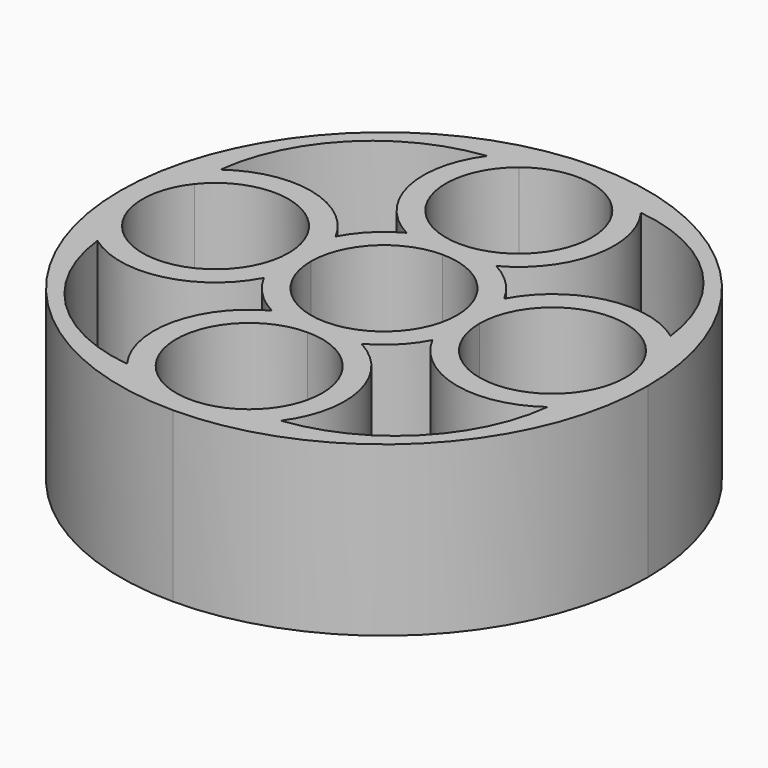
from build123d import *

# Parameters (mm, degrees)
F1_DEPTH = 25.4


# Not quite as in the source:
# - a feature names something its author has since deleted; it is built from what else it names


with BuildPart() as f1:
    # F0 (on Top) → F1 (new body)
    with BuildSketch(Plane.XY):
        with BuildLine():
            ThreePointArc((12.7, -6.7643328429), (11.4395600211, -3.4860169829), (11.0109, 0))
            ThreePointArc((11.0109, 0), (7.785882057, -7.785882057), (0, -11.0109))
            ThreePointArc((0, -11.0109), (3.4860169829, -11.4395600211), (6.7643328429, -12.7))
            ThreePointArc((6.7643328429, -12.7), (10.1746301852, -10.1746301852), (12.7, -6.7643328429))
        make_face()
        with BuildLine():
            ThreePointArc((-11.0109, 0), (-7.785882056, 7.7858820579), (2.7e-09, 11.0109))
            ThreePointArc((2.7e-09, 11.0109), (-3.4860169816, 11.4395600208), (-6.7643328429, 12.7))
            ThreePointArc((-6.7643328429, 12.7), (-10.1746301852, 10.1746301852), (-12.7, 6.7643328429))
            ThreePointArc((-12.7, 6.7643328429), (-11.4395600211, 3.4860169829), (-11.0109, 0))
        make_face()
        with BuildLine():
            ThreePointArc((6.7643328429, 12.7), (3.4860169842, 11.4395600214), (2.7e-09, 11.0109))
            ThreePointArc((2.7e-09, 11.0109), (7.7858820579, 7.785882056), (11.0109, 0))
            ThreePointArc((11.0109, 0), (11.4395600211, 3.4860169829), (12.7, 6.7643328429))
            ThreePointArc((12.7, 6.7643328429), (10.1746301852, 10.1746301852), (6.7643328429, 12.7))
        make_face()
        with BuildLine():
            ThreePointArc((0, -11.0109), (-7.785882057, -7.785882057), (-11.0109, 0))
            ThreePointArc((-11.0109, 0), (-11.4395600211, -3.4860169829), (-12.7, -6.7643328429))
            ThreePointArc((-12.7, -6.7643328429), (-10.1746301852, -10.1746301852), (-6.7643328429, -12.7))
            ThreePointArc((-6.7643328429, -12.7), (-3.4860169829, -11.4395600211), (0, -11.0109))
        make_face()
        with BuildLine():
            ThreePointArc((-6.8403930724, 34.02838), (0, 36.4109), (6.8403930724, 34.02838))
            ThreePointArc((6.8403930724, 34.02838), (9.216102766, 34.090951688), (11.5872617117, 33.9312112173))
            ThreePointArc((11.5872617117, 33.9312112173), (6.4919083282, 38.2413910878), (0, 39.7891))
            ThreePointArc((0, 39.7891), (-6.4919083282, 38.2413910878), (-11.5872617117, 33.9312112173))
            ThreePointArc((-11.5872617117, 33.9312112173), (-9.216102766, 34.090951688), (-6.8403930724, 34.02838))
        make_face()
        with BuildLine():
            ThreePointArc((0, 39.7891), (6.4919083282, 38.2413910878), (11.5872617117, 33.9312112173))
            ThreePointArc((11.5872617117, 33.9312112173), (26.6567838655, 26.6567838655), (33.9312112173, 11.5872617117))
            ThreePointArc((33.9312112173, 11.5872617117), (38.2413910878, 6.4919083282), (39.7891, 0))
            ThreePointArc((39.7891, 0), (28.1351424273, 28.1351424273), (0, 39.7891))
        make_face()
        with BuildLine():
            ThreePointArc((6.8403930724, 34.02838), (9.9135967966, 30.1917134059), (11.0109, 25.4))
            ThreePointArc((11.0109, 25.4), (7.7858820586, 17.6141179447), (4.7e-09, 14.3891))
            ThreePointArc((4.7e-09, 14.3891), (3.4860169852, 13.9604399783), (6.7643328429, 12.7))
            ThreePointArc((6.7643328429, 12.7), (12.3365080254, 17.9934644705), (14.3891, 25.4))
            ThreePointArc((14.3891, 25.4), (13.6707071197, 29.8897623163), (11.5872617117, 33.9312112173))
            ThreePointArc((11.5872617117, 33.9312112173), (9.216102766, 34.090951688), (6.8403930724, 34.02838))
        make_face()
        with BuildLine():
            ThreePointArc((-6.7643328429, 12.7), (-3.4860169806, 13.9604399795), (4.7e-09, 14.3891))
            ThreePointArc((4.7e-09, 14.3891), (-10.3982245629, 21.7782815197), (-6.8403930724, 34.02838))
            ThreePointArc((-6.8403930724, 34.02838), (-9.216102766, 34.090951688), (-11.5872617117, 33.9312112173))
            ThreePointArc((-11.5872617117, 33.9312112173), (-14.0316192263, 22.2125463616), (-6.7643328429, 12.7))
        make_face()
        with BuildLine():
            ThreePointArc((-33.9312112173, 11.5872617117), (-26.6567838655, 26.6567838655), (-11.5872617117, 33.9312112173))
            ThreePointArc((-11.5872617117, 33.9312112173), (-6.4919083282, 38.2413910878), (0, 39.7891))
            ThreePointArc((0, 39.7891), (-28.1351424273, 28.1351424273), (-39.7891, 0))
            ThreePointArc((-39.7891, 0), (-38.2413910878, 6.4919083282), (-33.9312112173, 11.5872617117))
        make_face()
        with BuildLine():
            ThreePointArc((-34.02838, 6.8403930724), (-34.090951688, 9.216102766), (-33.9312112173, 11.5872617117))
            ThreePointArc((-33.9312112173, 11.5872617117), (-38.2413910878, 6.4919083282), (-39.7891, 0))
            ThreePointArc((-39.7891, 0), (-38.2413910878, -6.4919083282), (-33.9312112173, -11.5872617117))
            ThreePointArc((-33.9312112173, -11.5872617117), (-34.090951688, -9.216102766), (-34.02838, -6.8403930724))
            ThreePointArc((-34.02838, -6.8403930724), (-36.4109, 0), (-34.02838, 6.8403930724))
        make_face()
        with BuildLine():
            ThreePointArc((-12.7, -6.7643328429), (-13.9604399789, -3.4860169829), (-14.3891, 0))
            ThreePointArc((-14.3891, 0), (-21.778281522, -10.3982245636), (-34.02838, -6.8403930724))
            ThreePointArc((-34.02838, -6.8403930724), (-34.090951688, -9.216102766), (-33.9312112173, -11.5872617117))
            ThreePointArc((-33.9312112173, -11.5872617117), (-22.2125463616, -14.0316192263), (-12.7, -6.7643328429))
        make_face()
        with BuildLine():
            ThreePointArc((-33.9312112173, -11.5872617117), (-38.2413910878, -6.4919083282), (-39.7891, 0))
            ThreePointArc((-39.7891, 0), (-28.1351424844, -28.1351423702), (-1.615e-07, -39.7891))
            ThreePointArc((-1.615e-07, -39.7891), (-6.4919084002, -38.2413910513), (-11.5872617117, -33.9312112173))
            ThreePointArc((-11.5872617117, -33.9312112173), (-26.6567838655, -26.6567838655), (-33.9312112173, -11.5872617117))
        make_face()
        with BuildLine():
            ThreePointArc((-6.8403930724, -34.02838), (-10.3982245667, -21.7782815309), (-1.89e-08, -14.3891))
            ThreePointArc((-1.89e-08, -14.3891), (-3.486016992, -13.9604399766), (-6.7643328429, -12.7))
            ThreePointArc((-6.7643328429, -12.7), (-14.0316192263, -22.2125463616), (-11.5872617117, -33.9312112173))
            ThreePointArc((-11.5872617117, -33.9312112173), (-9.216102766, -34.090951688), (-6.8403930724, -34.02838))
        make_face()
        with BuildLine():
            ThreePointArc((-11.5872617117, -33.9312112173), (-6.4919084002, -38.2413910513), (-1.615e-07, -39.7891))
            ThreePointArc((-1.615e-07, -39.7891), (6.4919082561, -38.2413911242), (11.5872617117, -33.9312112173))
            ThreePointArc((11.5872617117, -33.9312112173), (9.216102766, -34.090951688), (6.8403930724, -34.02838))
            ThreePointArc((6.8403930724, -34.02838), (0, -36.4109), (-6.8403930724, -34.02838))
            ThreePointArc((-6.8403930724, -34.02838), (-9.216102766, -34.090951688), (-11.5872617117, -33.9312112173))
        make_face()
        with BuildLine():
            ThreePointArc((6.7643328429, -12.7), (3.4860169737, -13.9604399812), (-1.89e-08, -14.3891))
            ThreePointArc((-1.89e-08, -14.3891), (7.7858820503, -17.6141179364), (11.0109, -25.4))
            ThreePointArc((11.0109, -25.4), (9.9135967966, -30.1917134059), (6.8403930724, -34.02838))
            ThreePointArc((6.8403930724, -34.02838), (9.216102766, -34.090951688), (11.5872617117, -33.9312112173))
            ThreePointArc((11.5872617117, -33.9312112173), (13.6707071197, -29.8897623163), (14.3891, -25.4))
            ThreePointArc((14.3891, -25.4), (12.3365080254, -17.9934644705), (6.7643328429, -12.7))
        make_face()
        with BuildLine():
            ThreePointArc((-1.615e-07, -39.7891), (28.1351423702, -28.1351424844), (39.7891, 0))
            ThreePointArc((39.7891, 0), (38.2413910878, -6.4919083282), (33.9312112173, -11.5872617117))
            ThreePointArc((33.9312112173, -11.5872617117), (26.6567838655, -26.6567838655), (11.5872617117, -33.9312112173))
            ThreePointArc((11.5872617117, -33.9312112173), (6.4919082561, -38.2413911242), (-1.615e-07, -39.7891))
        make_face()
        with BuildLine():
            ThreePointArc((39.7891, 0), (38.2413910878, 6.4919083282), (33.9312112173, 11.5872617117))
            ThreePointArc((33.9312112173, 11.5872617117), (34.090951688, 9.216102766), (34.02838, 6.8403930724))
            ThreePointArc((34.02838, 6.8403930724), (35.7982245636, 3.621718478), (36.4109, 0))
            ThreePointArc((36.4109, 0), (35.7982245636, -3.621718478), (34.02838, -6.8403930724))
            ThreePointArc((34.02838, -6.8403930724), (34.090951688, -9.216102766), (33.9312112173, -11.5872617117))
            ThreePointArc((33.9312112173, -11.5872617117), (38.2413910878, -6.4919083282), (39.7891, 0))
        make_face()
        with BuildLine():
            ThreePointArc((34.02838, 6.8403930724), (34.090951688, 9.216102766), (33.9312112173, 11.5872617117))
            ThreePointArc((33.9312112173, 11.5872617117), (22.2125463616, 14.0316192263), (12.7, 6.7643328429))
            ThreePointArc((12.7, 6.7643328429), (13.9604399789, 3.4860169829), (14.3891, 0))
            ThreePointArc((14.3891, 0), (21.778281522, 10.3982245636), (34.02838, 6.8403930724))
        make_face()
        with BuildLine():
            ThreePointArc((12.7, 6.7643328429), (11.4395600211, 3.4860169829), (11.0109, 0))
            Line((11.0109, 0), (14.3891, 0))
            ThreePointArc((14.3891, 0), (13.9604399789, 3.4860169829), (12.7, 6.7643328429))
        make_face()
        with BuildLine():
            Line((14.3891, 0), (11.0109, 0))
            ThreePointArc((11.0109, 0), (11.4395600211, -3.4860169829), (12.7, -6.7643328429))
            ThreePointArc((12.7, -6.7643328429), (13.9604399789, -3.4860169829), (14.3891, 0))
        make_face()
        with BuildLine():
            ThreePointArc((34.02838, -6.8403930724), (21.778281522, -10.3982245636), (14.3891, 0))
            ThreePointArc((14.3891, 0), (13.9604399789, -3.4860169829), (12.7, -6.7643328429))
            ThreePointArc((12.7, -6.7643328429), (22.2125463616, -14.0316192263), (33.9312112173, -11.5872617117))
            ThreePointArc((33.9312112173, -11.5872617117), (34.090951688, -9.216102766), (34.02838, -6.8403930724))
        make_face()
        with BuildLine():
            ThreePointArc((6.7643328429, -12.7), (3.4860169829, -11.4395600211), (0, -11.0109))
            Line((0, -11.0109), (0, -14.3891))
            ThreePointArc((-1.89e-08, -14.3891), (3.4860169737, -13.9604399812), (6.7643328429, -12.7))
        make_face()
        with BuildLine():
            Line((0, -14.3891), (0, -11.0109))
            ThreePointArc((0, -11.0109), (-3.4860169829, -11.4395600211), (-6.7643328429, -12.7))
            ThreePointArc((-6.7643328429, -12.7), (-3.486016992, -13.9604399766), (-1.89e-08, -14.3891))
        make_face()
        with BuildLine():
            ThreePointArc((-12.7, -6.7643328429), (-11.4395600211, -3.4860169829), (-11.0109, 0))
            Line((-11.0109, 0), (-14.3891, 0))
            ThreePointArc((-14.3891, 0), (-13.9604399789, -3.4860169829), (-12.7, -6.7643328429))
        make_face()
        with BuildLine():
            Line((-14.3891, 0), (-11.0109, 0))
            ThreePointArc((-11.0109, 0), (-11.4395600211, 3.4860169829), (-12.7, 6.7643328429))
            ThreePointArc((-12.7, 6.7643328429), (-13.9604399789, 3.4860169829), (-14.3891, 0))
        make_face()
        with BuildLine():
            Line((0, 11.0109), (0, 14.3891))
            ThreePointArc((4.7e-09, 14.3891), (-3.4860169806, 13.9604399795), (-6.7643328429, 12.7))
            ThreePointArc((-6.7643328429, 12.7), (-3.4860169816, 11.4395600208), (2.7e-09, 11.0109))
        make_face()
        with BuildLine():
            ThreePointArc((6.7643328429, 12.7), (3.4860169852, 13.9604399783), (4.7e-09, 14.3891))
            Line((0, 14.3891), (0, 11.0109))
            ThreePointArc((2.7e-09, 11.0109), (3.4860169842, 11.4395600214), (6.7643328429, 12.7))
        make_face()
        with BuildLine():
            ThreePointArc((-14.3891, 0), (-13.9604399789, 3.4860169829), (-12.7, 6.7643328429))
            ThreePointArc((-12.7, 6.7643328429), (-22.2125463616, 14.0316192263), (-33.9312112173, 11.5872617117))
            ThreePointArc((-33.9312112173, 11.5872617117), (-34.090951688, 9.216102766), (-34.02838, 6.8403930724))
            ThreePointArc((-34.02838, 6.8403930724), (-21.778281522, 10.3982245636), (-14.3891, 0))
        make_face()
    extrude(amount=F1_DEPTH)


solid = f1.part
